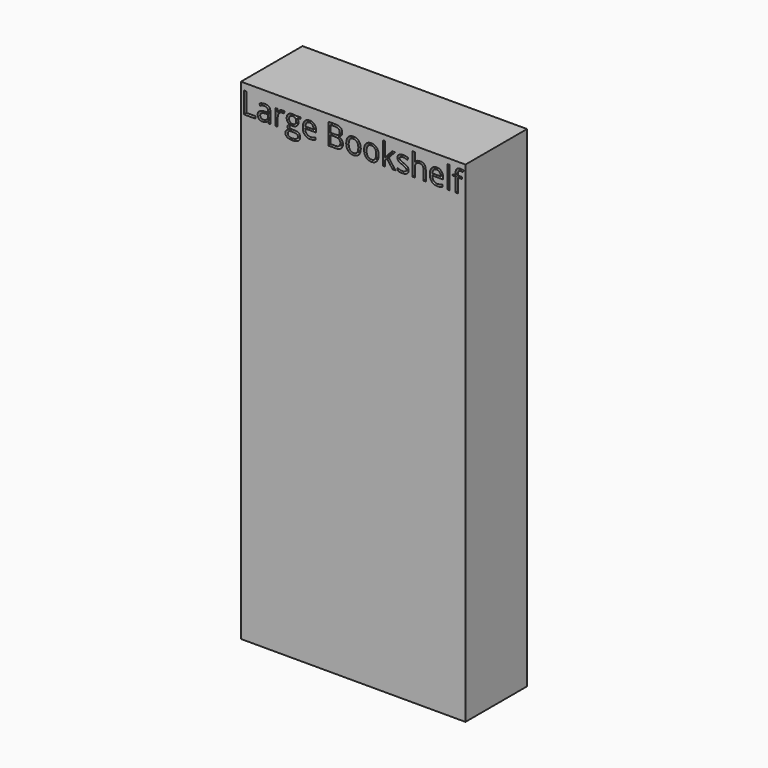
from build123d import *

# Parameters (mm, degrees)
F0_W         = 889
F0_H         = 1943.1
F1_DEPTH     = 152.4
F2_TEXT_SIZE = 117.2098389024
F3_DEPTH     = 25.4


# Not quite as in the source:
# - Text() gives the source's letters only with a copy of the font that has no kerning and outlines rounded to 1/6400 em; it was checked with that copy


with BuildPart() as f1:
    # F0 (on Front) → F1 (new body, symmetric)
    with BuildSketch(Plane.XZ):
        Rectangle(F0_W, F0_H)
    extrude(amount=F1_DEPTH, both=True)

    # F2 (on face) → F3 (cut)
    with BuildSketch(Plane.XZ.offset(152.4)):
        with Locations((-444.5, 860.9869337019)):
            Text('Large Bookshelf', F2_TEXT_SIZE, font='Open Sans', text_align=(TextAlign.LEFT, TextAlign.BOTTOM))
    extrude(amount=-F3_DEPTH, mode=Mode.SUBTRACT)


solid = f1.part
